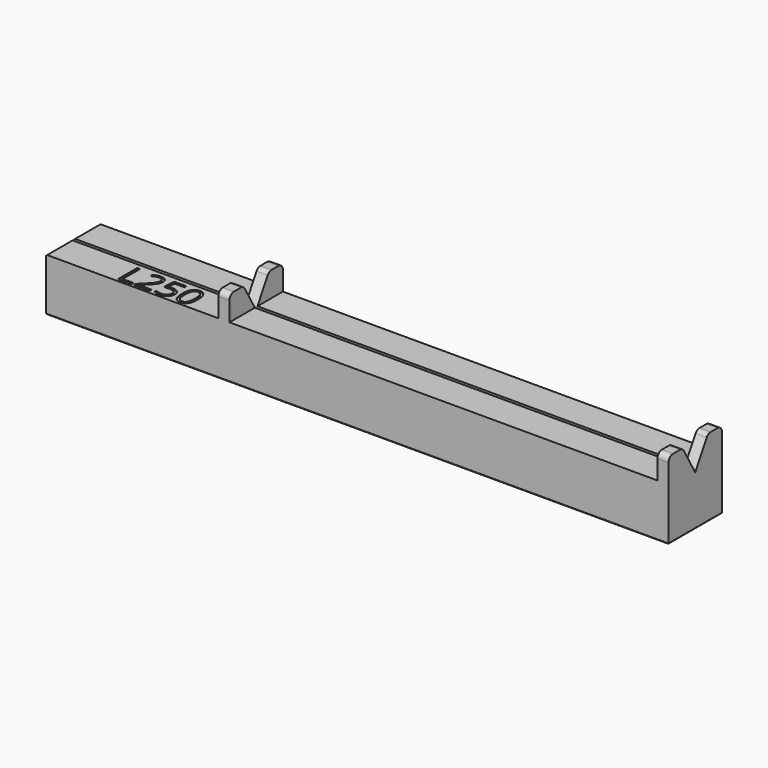
from build123d import *

# Parameters (mm, degrees)
F0_W         = 56
F0_H         = 6
F1_DEPTH     = 7
F2_W         = 38.5
F2_H         = 6
F2_W_2       = 15.5
F3_DEPTH     = 2.237
F5_DEPTH     = 56.001
F6_R         = 0.5
F7_SIZE      = 0.1
F8_TEXT_SIZE = 3.0347208344
F9_DEPTH     = 0.1


# Not quite as in the source:
# - Text() gives the source's letters only with a copy of the font that has no kerning and outlines rounded to 1/6400 em; it was checked with that copy


with BuildPart() as f1:
    # F0 (on Top) → F1 (new body)
    with BuildSketch(Plane.XY):
        Rectangle(F0_W, F0_H)
    extrude(amount=F1_DEPTH)

    # F2 (on face) → F3 (cut)
    with BuildSketch(Plane.XY.offset(7)):
        with Locations((7.75, 0)):
            Rectangle(F2_W, F2_H)
        with Locations((-20.25, 0)):
            Rectangle(F2_W_2, F2_H)
    extrude(amount=-F3_DEPTH, mode=Mode.SUBTRACT)

    # F4 (on face) → F5 (cut, through all)
    with BuildSketch(Plane.YZ.offset(28)):
        with BuildLine():
            Line((1.4372579996, 7), (-1.4372579996, 7))
            Line((-1.4372579996, 7), (-0.1093523805, 4.7))
            Line((-0.1093523805, 4.7), (-0.0461939766, 4.5475221249))
            ThreePointArc((-0.0461939766, 4.5475221249), (0, 4.5166562965), (0.0461939766, 4.5475221249))
            Line((0.0461939766, 4.5475221249), (0.1093523805, 4.7))
            Line((0.1093523805, 4.7), (1.4372579996, 7))
        make_face()
    extrude(amount=-F5_DEPTH, mode=Mode.SUBTRACT)

    # F6
    f6_edges = [f1.edges().sort_by_distance(p)[0] for p in [
        (27.5, -3, 7),
        (27.5, 3, 7),
        (-12, -3, 7),
        (-12, 3, 7),
        (-12, 1.437258, 7),
        (-12, -1.437258, 7),
        (27.5, -1.437258, 7),
        (27.5, 1.437258, 7),
    ]]
    fillet(f6_edges, radius=F6_R)

    # F7
    f7_edges = [f1.edges().sort_by_distance(p)[0] for p in [
        (0, -3, 0),
        (28, 0, 0),
        (0, 3, 0),
        (-28, 0, 0),
        (-28, -1.572863, 4.763),
        (-28, 1.572863, 4.763),
    ]]
    chamfer(f7_edges, length=F7_SIZE)

    # F8 (on face) → F9 (cut)
    with BuildSketch(Plane.XY.offset(4.763)):
        with Locations((-22.0286250114, -2.7570896782)):
            Text('L250', F8_TEXT_SIZE, font='Open Sans', text_align=(TextAlign.LEFT, TextAlign.BOTTOM))
    extrude(amount=-F9_DEPTH, mode=Mode.SUBTRACT)


solid = f1.part
